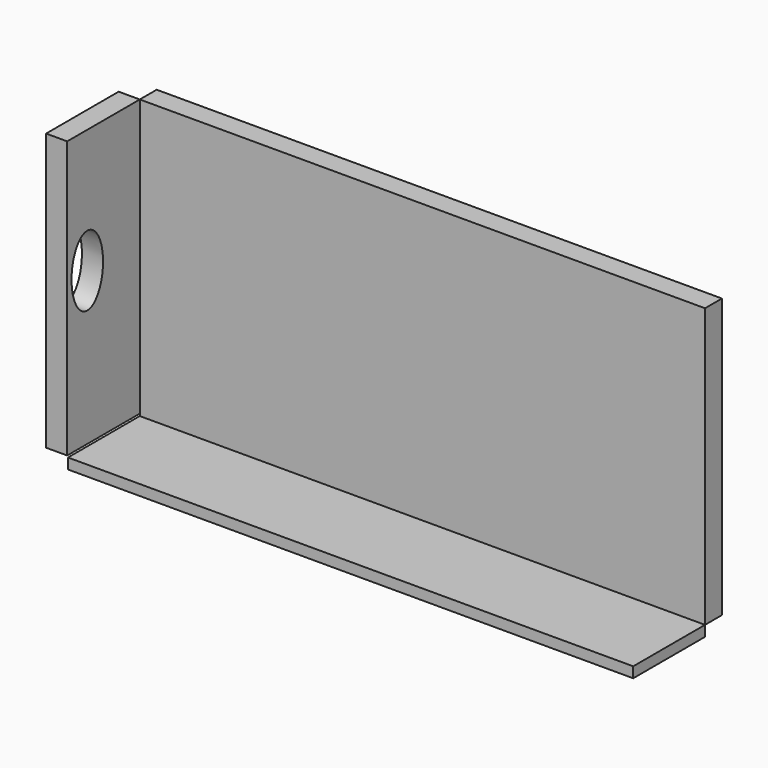
from build123d import *

# Parameters (mm, degrees)
F0_W     = 135.9073966742
F0_H     = 67.0142434537
F1_DEPTH = 5.08
F2_W     = 21.8143142146
F2_H     = 66.5003098547
F3_DEPTH = 5.08
F5_W     = 135.9073966742
F5_H     = 21.5824521464
F6_DEPTH = 2.54


# Not quite as in the source:
# - the program builds the solid bodies; features that only make, move or delete a surface that nothing else refers to are left out


with BuildPart() as f1:
    # F0 (on Front) → F1 (new body)
    with BuildSketch(Plane.XZ):
        with Locations((-2.3486316204, -0.1565758139)):
            Rectangle(F0_W, F0_H)
    extrude(amount=F1_DEPTH)


with BuildPart() as f3:
    # F2 (on face) → F3 (new body)
    with BuildSketch(Plane(origin=(-70.3023299575, 0, 0), x_dir=(0, -1, 0), z_dir=(-1, 0, 0))):
        with Locations((15.9871571073, 0.1003909856)):
            Rectangle(F2_W, F2_H)
        with BuildLine():
            add(Edge.make_bspline(
                [(20.860183984, -4.9150027335), (29.0597432151, -4.9150027335), (24.9599635996, 7.7609560685), (20.860183984, 20.4369148705), (16.7604043685, 7.7609560685), (12.6606247529, -4.9150027335), (20.860183984, -4.9150027335)],
                knots=[0, 0, 0, 2.0943951024, 2.0943951024, 4.1887902048, 4.1887902048, 6.2831853072, 6.2831853072, 6.2831853072], degree=2, weights=[1, 0.5, 1, 0.5, 1, 0.5, 1]))
        make_face(mode=Mode.SUBTRACT)
    extrude(amount=F3_DEPTH)


with BuildPart() as f6:
    # F5 (on face) → F6 (new body)
    with BuildSketch(Plane(origin=(0, 0, -33.6636975408), x_dir=(1, 0, 0), z_dir=(0, 0, -1))):
        with Locations((-2.3486316204, 15.8712260732)):
            Rectangle(F5_W, F5_H)
    extrude(amount=F6_DEPTH)


solid = Compound([f1.part, f3.part, f6.part])
